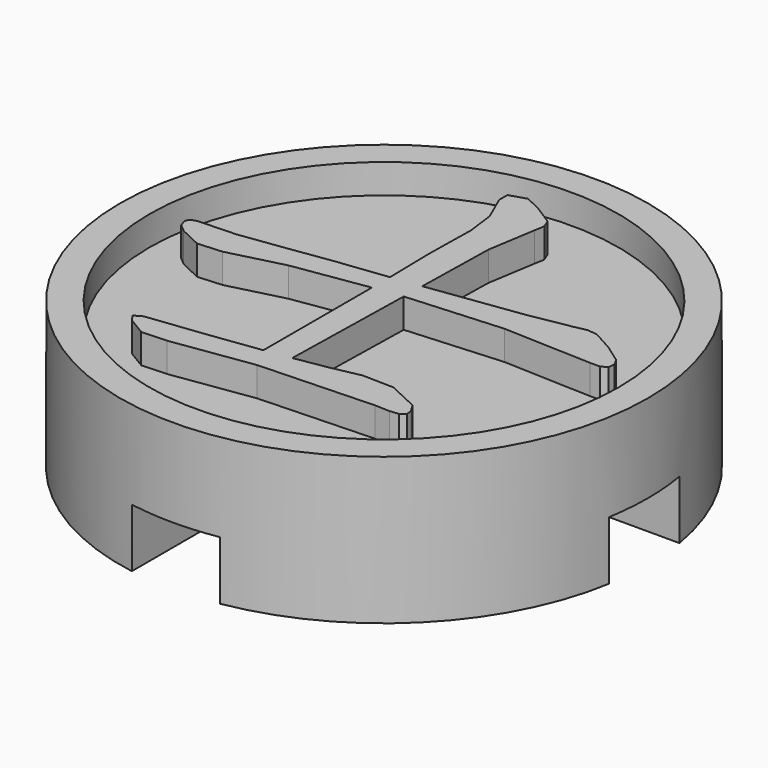
from build123d import *

# Parameters (mm, degrees)
F0_R     = 9
F1_DEPTH = 4
F3_W     = 3
F3_H     = 3
F4_DEPTH = 2
F2_R     = 9
F2_R_2   = 8
F5_DEPTH = 1
F7_DEPTH = 1


# Not quite as in the source:
# - a feature names something its author has since deleted; it is built from what else it names


with BuildPart() as f1:
    # F0 (on Top) → F1 (new body)
    with BuildSketch(Plane.XY):
        with Locations((-31.3306450844, 19.7580661625)):
            Circle(F0_R)
    extrude(amount=F1_DEPTH)

    # F3 (on face) → F4 (cut)
    with BuildSketch(Plane(origin=(0, 0, 0), x_dir=(1, 0, 0), z_dir=(0, 0, -1))):
        with BuildLine():
            ThreePointArc((-32.8306450844, -28.6321858371), (-32.0832814269, -28.7265408676), (-31.3306450844, -28.7580661625))
            ThreePointArc((-31.3306450844, -28.7580661625), (-30.5780087419, -28.7265408676), (-29.8306450844, -28.6321858371))
            Line((-29.8306450844, -28.6321858371), (-29.8306450844, -21.2580661625))
            Line((-29.8306450844, -21.2580661625), (-32.8306450844, -21.2580661625))
            Line((-32.8306450844, -21.2580661625), (-32.8306450844, -28.6321858371))
        make_face()
        with BuildLine():
            ThreePointArc((-40.204764759, -18.2580661625), (-40.2991197895, -19.0054298199), (-40.3306450844, -19.7580661625))
            ThreePointArc((-40.3306450844, -19.7580661625), (-40.2991197895, -20.510702505), (-40.204764759, -21.2580661625))
            Line((-40.204764759, -21.2580661625), (-32.8306450844, -21.2580661625))
            Line((-32.8306450844, -21.2580661625), (-32.8306450844, -18.2580661625))
            Line((-32.8306450844, -18.2580661625), (-40.204764759, -18.2580661625))
        make_face()
        with Locations((-31.3306450844, -19.7580661625)):
            Rectangle(F3_W, F3_H)
        with BuildLine():
            Line((-29.8306450844, -18.2580661625), (-29.8306450844, -21.2580661625))
            Line((-29.8306450844, -21.2580661625), (-22.4565254097, -21.2580661625))
            ThreePointArc((-22.4565254097, -21.2580661625), (-22.3621703793, -20.510702505), (-22.3306450844, -19.7580661625))
            ThreePointArc((-22.3306450844, -19.7580661625), (-22.3621703793, -19.0054298199), (-22.4565254097, -18.2580661625))
            Line((-22.4565254097, -18.2580661625), (-29.8306450844, -18.2580661625))
        make_face()
        with BuildLine():
            Line((-32.8306450844, -10.8839464878), (-32.8306450844, -18.2580661625))
            Line((-32.8306450844, -18.2580661625), (-29.8306450844, -18.2580661625))
            Line((-29.8306450844, -18.2580661625), (-29.8306450844, -10.8839464878))
            ThreePointArc((-29.8306450844, -10.8839464878), (-30.5780087419, -10.7895914574), (-31.3306450844, -10.7580661625))
            ThreePointArc((-31.3306450844, -10.7580661625), (-32.0832814269, -10.7895914574), (-32.8306450844, -10.8839464878))
        make_face()
    extrude(amount=-F4_DEPTH, mode=Mode.SUBTRACT)

    # F2 (on face) → F5 (join)
    with BuildSketch(Plane.XY.offset(4)):
        with Locations((-31.3306450844, 19.7580661625)):
            Circle(F2_R)
        with Locations((-31.3306450844, 19.7580661625)):
            Circle(F2_R_2, mode=Mode.SUBTRACT)
    extrude(amount=F5_DEPTH)

    # F6 (on face) → F7 (join)
    with BuildSketch(Plane.XY.offset(4)):
        Polygon((-32.0563357805, 20.1492391588), (-32.0563357805, 15.5241883096), (-33.8901808177, 15.2807091812), (-35.7654903866, 15.0600261471), (-36.0265778437, 14.9108290182), (-35.8773882333, 14.6911827853), (-35.2526459317, 14.3130134752), (-34.3978675811, 14.3513488068), (-31.6491488168, 14.7523119557), (-27.7544977602, 14.8984009364), (-27.2406082337, 14.8818211386), (-26.9360337682, 14.9129041244), (-26.7764911822, 15.0434478529), (-26.7972422443, 15.2371920988), (-26.9670851763, 15.5241883096), (-28.0156152913, 16.0142517072), (-29.0890316438, 16.0380853546), (-30.0566626908, 15.8391533431), (-31.1736036441, 15.6526644505), (-31.0741413977, 20.2777152997), (-27.8239687071, 20.5025335092), (-24.8161924809, 20.3896206649), (-24.4701910762, 20.3927258057), (-24.2691463661, 20.5014959561), (-24.248470489, 20.7273742743), (-24.368616131, 20.9532450739), (-25.0037038896, 21.403934083), (-25.6989396543, 21.7862799203), (-26.0398284784, 21.8225190939), (-26.4241742369, 21.7406426207), (-27.8850941182, 21.4816227513), (-31.057540548, 21.0485495894), (-31.0016029024, 23.7941707314), (-30.738440339, 25.4290687202), (-30.678367518, 25.7761979), (-30.788137629, 26.0549087229), (-31.4533219461, 26.4797040154), (-32.0066084166, 26.7469867172), (-32.5702328255, 26.5687982493), (-32.5702328255, 26.2164813041), (-32.1775490497, 25.3202760143), (-32.0563357805, 24.3681330789), (-32.0874247812, 22.6793274398), (-32.0563357805, 20.9200960041), (-33.8093644531, 20.709758427), (-35.2516083786, 20.5014959561), (-36.7901718172, 20.2932635593), (-38.0780173149, 20.2445662299), (-38.2831611116, 20.1761854655), (-38.351541876, 20.0373337936), (-38.2738359152, 19.7938772208), (-38.0117086494, 19.5731716311), (-37.2781676271, 19.2260875624), (-36.4534482425, 19.2830853166), (-34.5957620394, 19.7586530447), align=None)
    extrude(amount=F7_DEPTH)


solid = f1.part
